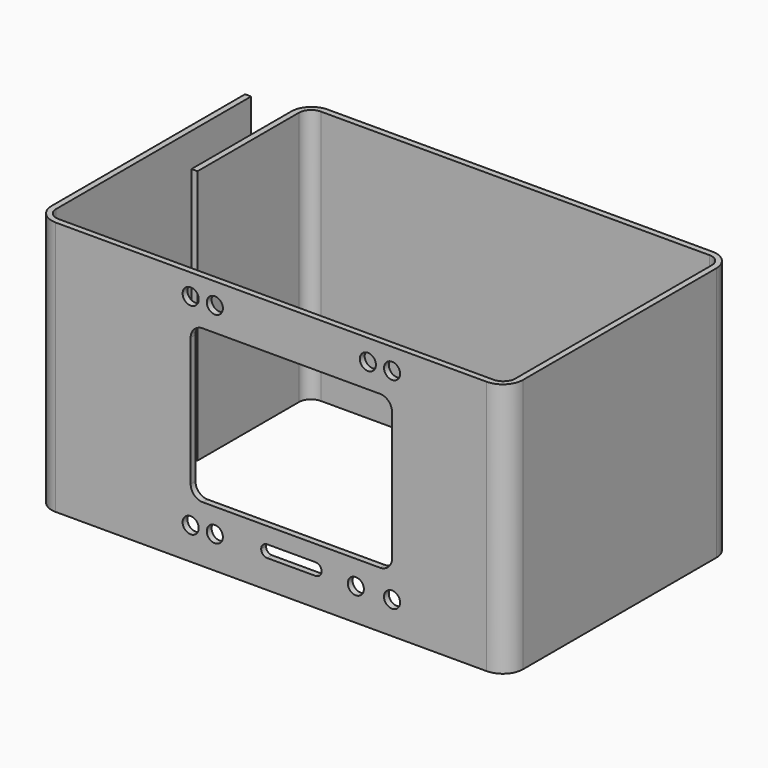
from build123d import *

# Parameters (mm, degrees)
F1_DEPTH = 63.25
F2_R     = 2
F3_DEPTH = 25


# Not quite as in the source:
# - a feature names something its author has since deleted; it is built from what else it names


with BuildPart() as f1:
    # F0 (on Top) → F1 (new body)
    with BuildSketch(Plane.XY):
        with BuildLine():
            Line((-62.75, -30.5), (-62.75, 30))
            Line((-62.75, 30), (-64.25, 30))
            Line((-64.25, 30), (-64.25, -30))
            ThreePointArc((-64.25, -30), (-62.7855339059, -33.5355339059), (-59.25, -35))
            Line((-59.25, -35), (47.75, -35))
            ThreePointArc((47.75, -35), (51.2855339059, -33.5355339059), (52.75, -30))
            Line((52.75, -30), (52.75, 30))
            ThreePointArc((52.75, 30), (51.2855339059, 33.5355339059), (47.75, 35))
            Line((47.75, 35), (-47.75, 35))
            ThreePointArc((-47.75, 35), (-51.2855339059, 33.5355339059), (-52.75, 30))
            Line((-52.75, 30), (-52.75, -1))
            Line((-52.75, -1), (-51.25, -1))
            Line((-51.25, -1), (-51.25, 30.5))
            ThreePointArc((-51.25, 30.5), (-50.3713203436, 32.6213203436), (-48.25, 33.5))
            Line((-48.25, 33.5), (48.25, 33.5))
            ThreePointArc((48.25, 33.5), (50.3713203436, 32.6213203436), (51.25, 30.5))
            Line((51.25, 30.5), (51.25, -30.5))
            ThreePointArc((51.25, -30.5), (50.3713203436, -32.6213203436), (48.25, -33.5))
            Line((48.25, -33.5), (-59.75, -33.5))
            ThreePointArc((-59.75, -33.5), (-61.8713203436, -32.6213203436), (-62.75, -30.5))
        make_face()
    extrude(amount=F1_DEPTH)

    # F2 (on face) → F3 (cut)
    with BuildSketch(Plane.XZ.offset(35)):
        with BuildLine():
            Line((21.25, 52), (-22.75, 52))
            ThreePointArc((-22.75, 52), (-24.8713203436, 51.1213203436), (-25.75, 49))
            Line((-25.75, 49), (-25.75, 17))
            ThreePointArc((-25.75, 17), (-24.8713203436, 14.8786796564), (-22.75, 14))
            Line((-22.75, 14), (21.25, 14))
            ThreePointArc((21.25, 14), (23.3713203436, 14.8786796564), (24.25, 17))
            Line((24.25, 17), (24.25, 49))
            ThreePointArc((24.25, 49), (23.3713203436, 51.1213203436), (21.25, 52))
        make_face()
        with Locations((-25.75, 58)):
            Circle(F2_R)
        with Locations((24.25, 58)):
            Circle(F2_R)
        with Locations((24.25, 8)):
            Circle(F2_R)
        with Locations((-25.75, 8)):
            Circle(F2_R)
        with BuildLine():
            ThreePointArc((-8.25, 8.5), (-7.8106601718, 7.4393398282), (-6.75, 7))
            Line((-6.75, 7), (5.25, 7))
            ThreePointArc((5.25, 7), (6.3106601718, 7.4393398282), (6.75, 8.5))
            ThreePointArc((6.75, 8.5), (6.3106601718, 9.5606601718), (5.25, 10))
            Line((5.25, 10), (-6.75, 10))
            ThreePointArc((-6.75, 10), (-7.8106601718, 9.5606601718), (-8.25, 8.5))
        make_face()
        with Locations((-19.75, 8)):
            Circle(F2_R)
        with Locations((-19.75, 58)):
            Circle(F2_R)
        with Locations((18.25, 58)):
            Circle(F2_R)
        with Locations((15.25, 8)):
            Circle(F2_R)
    extrude(amount=-F3_DEPTH, mode=Mode.SUBTRACT)


solid = f1.part
